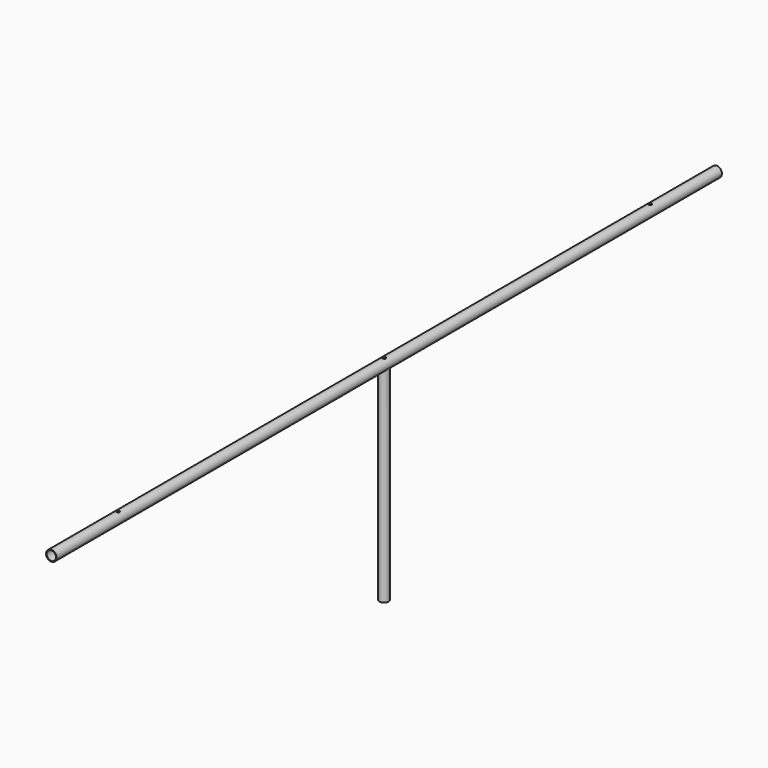
from build123d import *

# Parameters (mm, degrees)
F0_R     = 12.7
F0_R_2   = 11.2
F1_DEPTH = 1000
F2_R     = 11.2
F2_R_2   = 10
F3_DEPTH = 500
F4_R     = 12.7
F5_DEPTH = 12.5
F6_R     = 4
F7_DEPTH = 15


with BuildPart() as f1:
    # F0 (on Front) → F1 (new body, symmetric)
    with BuildSketch(Plane.XZ):
        Circle(F0_R)
        Circle(F0_R_2, mode=Mode.SUBTRACT)
    extrude(amount=F1_DEPTH, both=True)

    # F6 (on Top) → F7 (cut, symmetric)
    with BuildSketch(Plane.XY):
        Circle(F6_R)
        with Locations((0, 800)):
            Circle(F6_R)
        with Locations((0, -800)):
            Circle(F6_R)
    extrude(amount=F7_DEPTH, both=True, mode=Mode.SUBTRACT)


with BuildPart() as f3:
    # F2 (on Top) → F3 (new body)
    with BuildSketch(Plane.XY):
        Circle(F2_R)
        Circle(F2_R_2, mode=Mode.SUBTRACT)
    extrude(amount=-F3_DEPTH)

    # F4 (on Front) → F5 (cut, symmetric)
    with BuildSketch(Plane.XZ):
        Circle(F4_R)
    extrude(amount=F5_DEPTH, both=True, mode=Mode.SUBTRACT)


solid = Compound([f1.part, f3.part])
